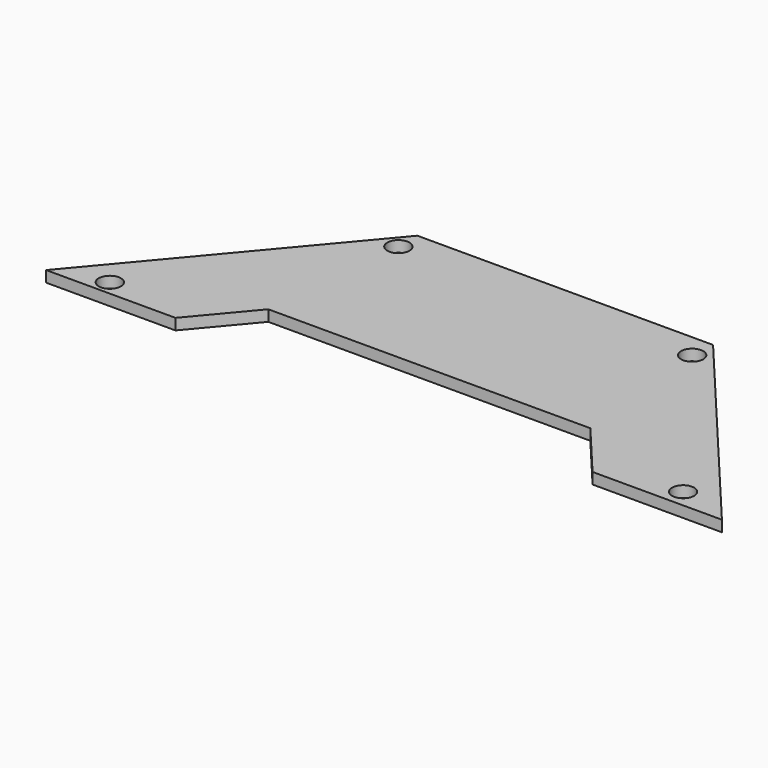
from build123d import *

# Parameters (mm, degrees)
F0_R     = 19.05
F1_DEPTH = 19.05


# Not quite as in the source:
# - the program builds the solid bodies; features that only make, move or delete a surface that nothing else refers to are left out


with BuildPart() as f1:
    # F0 (on Top) → F1 (new body)
    with BuildSketch(Plane.XY):
        Polygon((579.6451972242, -389.1505771044), (253.1090915034, 0), (-254.8909084966, 0), (-581.4270142173, -389.1505771044), (-359.1770142173, -389.1505771044), (-277.5429877872, -291.8629328283), (275.761170794, -291.8629328283), (357.3951972242, -389.1505771044), align=None)
        with Locations((-492.4777746201, -363.489061594)):
            Circle(F0_R, mode=Mode.SUBTRACT)
        with Locations((488.1779849529, -358.251363039)):
            Circle(F0_R, mode=Mode.SUBTRACT)
        with Locations((-254.8909084966, -40.7918766141)):
            Circle(F0_R, mode=Mode.SUBTRACT)
        with Locations((249.8159110546, -40.7918766141)):
            Circle(F0_R, mode=Mode.SUBTRACT)
    extrude(amount=F1_DEPTH)


solid = f1.part
